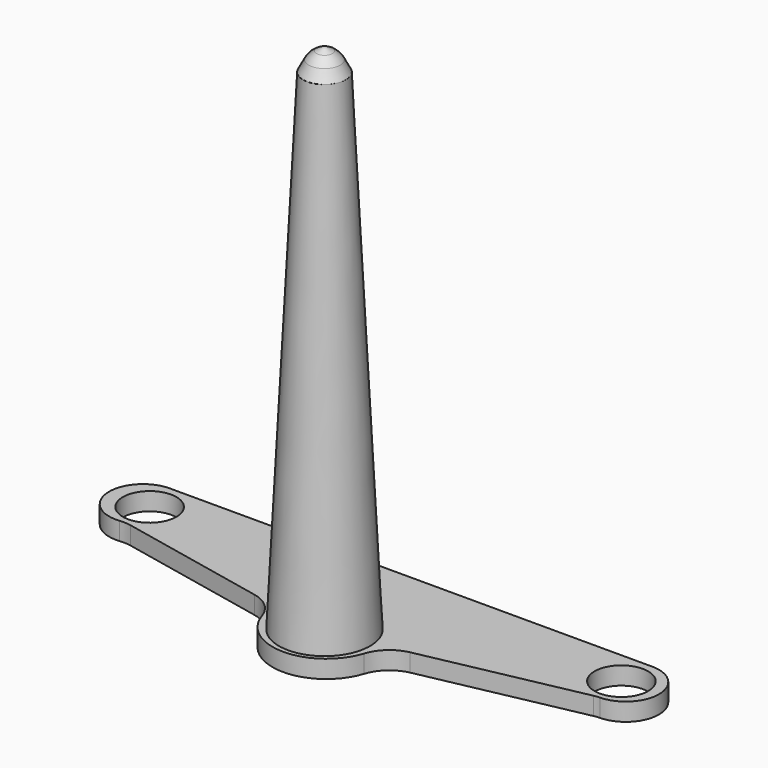
from build123d import *

# Parameters (mm, degrees)
F0_R     = 2.25
F0_R_2   = 1.5
F1_DEPTH = 1
F2_R     = 2
F5_R     = 2
F6_DEPTH = 29.7303643356
F6_TAPER = 4
F7_R     = 1


with BuildPart() as f1:
    # F0 (on Top) → F1 (new body)
    with BuildSketch(Plane.XY):
        with BuildLine():
            Line((13.3969206363, 1.9189893501), (-13.6030793637, 1.9189893501))
            ThreePointArc((-13.6030793637, 1.9189893501), (-15.476354869, -0.2010418621), (-13.1418243737, -1.7990596423))
            Line((-13.1418243737, -1.7990596423), (-3.0734528816, -3.9087251454))
            ThreePointArc((-3.0734528816, -3.9087251454), (-0.0744018388, -7.0627152846), (2.9271771184, -3.9111308071))
            Line((2.9271771184, -3.9111308071), (13.3021756263, -1.7970976995))
            ThreePointArc((13.3021756263, -1.7970976995), (15.2555679655, 0.0123501208), (13.3969206363, 1.9189893501))
        make_face()
        with Locations((0, -4.3)):
            Circle(F0_R, mode=Mode.SUBTRACT)
        with Locations((-13.2, 0)):
            Circle(F0_R_2, mode=Mode.SUBTRACT)
        with Locations((13.2, 0)):
            Circle(F0_R_2, mode=Mode.SUBTRACT)
    extrude(amount=F1_DEPTH)

    # F2
    f2_edges = [f1.edges().sort_by_distance(p)[0] for p in [
        (2.927177, -3.911131, 0.5),
        (13.302176, -1.797098, 0.5),
        (-13.141824, -1.79906, 0.5),
        (-3.073453, -3.908725, 0.5),
    ]]
    fillet(f2_edges, radius=F2_R)

    # F3 (on Right) → F4 (revolve)
    with BuildSketch(Plane.YZ):
        Polygon((-4.2690001428, 0), (-1.6726437025, 0), (-3.0743933748, 28.4580495209), (-3.5435410682, 29.3574947864), (-4.2690001428, 29.7293643356), align=None)
    revolve(axis=Axis((0, -4.2690001428, 17.7293643356), (0, 0, 1)))

    # F5 (on face) → F6 (cut, through all)
    with BuildSketch(Plane.XY):
        with Locations((0, -4.2691347189)):
            Circle(F5_R)
    extrude(amount=F6_DEPTH, taper=F6_TAPER, mode=Mode.SUBTRACT)

    # F7
    f7_edges = [f1.edges().sort_by_distance(p)[0] for p in [
        (0, -4.994459, 29.357495),
    ]]
    fillet(f7_edges, radius=F7_R)


solid = f1.part
